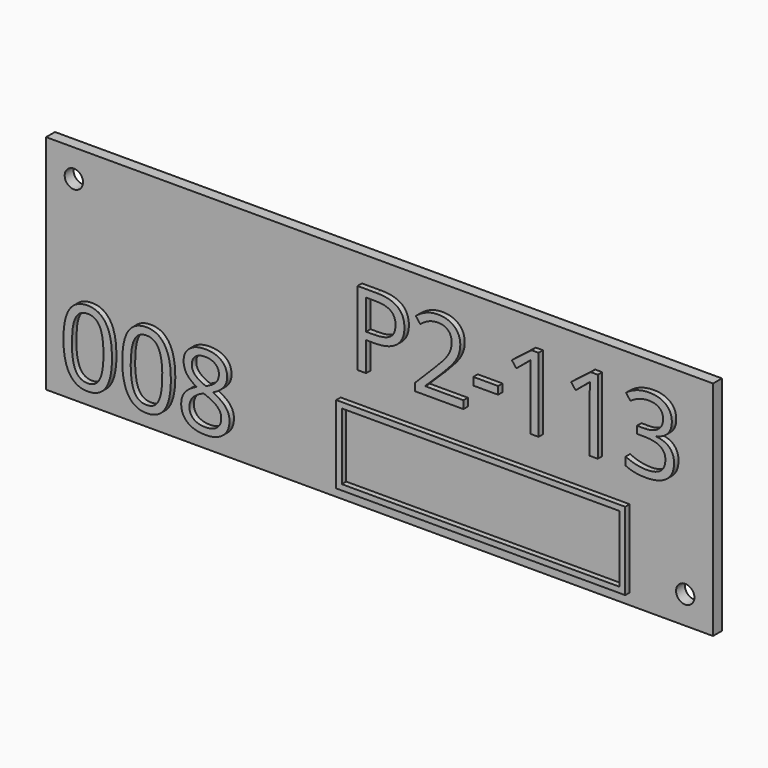
from build123d import *

# Parameters (mm, degrees)
F0_W         = 120
F0_H         = 40
F1_DEPTH     = 2
F3_D         = 3.3
F4_TEXT_SIZE = 18.651641733
F5_DEPTH     = 1
F6_TEXT_SIZE = 18.5155049272
F7_DEPTH     = 1
F8_W         = 52
F8_H         = 14
F8_W_2       = 49.99999962
F8_H_2       = 11.99999962
F9_DEPTH     = 1


# Not quite as in the source:
# - Text() gives the source's letters only with a copy of the font that has no kerning and outlines rounded to 1/6400 em; it was checked with that copy


with BuildPart() as f1:
    # F0 (on Front) → F1 (new body)
    with BuildSketch(Plane.XZ):
        Rectangle(F0_W, F0_H)
    extrude(amount=F1_DEPTH)

    # F3 (through all)
    with Locations(Plane.XZ.offset(2)):
        with Locations((-55, 15), (55, -15)):
            Hole(F3_D / 2)

    # F4 (on face) → F5 (join)
    with BuildSketch(Plane.XZ.offset(2)):
        with Locations((-5, 2)):
            Text('P2-113', F4_TEXT_SIZE, font='Open Sans', text_align=(TextAlign.LEFT, TextAlign.BOTTOM))
    extrude(amount=F5_DEPTH)

    # F6 (on face) → F7 (join)
    with BuildSketch(Plane.XZ.offset(2)):
        with Locations((-57, -17)):
            Text('008', F6_TEXT_SIZE, font='Open Sans', text_align=(TextAlign.LEFT, TextAlign.BOTTOM))
    extrude(amount=F7_DEPTH)

    # F8 (on face) → F9 (join)
    with BuildSketch(Plane.XZ.offset(2)):
        with Locations((19, -11)):
            Rectangle(F8_W, F8_H)
        with Locations((19, -11)):
            Rectangle(F8_W_2, F8_H_2, mode=Mode.SUBTRACT)
    extrude(amount=F9_DEPTH)


solid = f1.part
